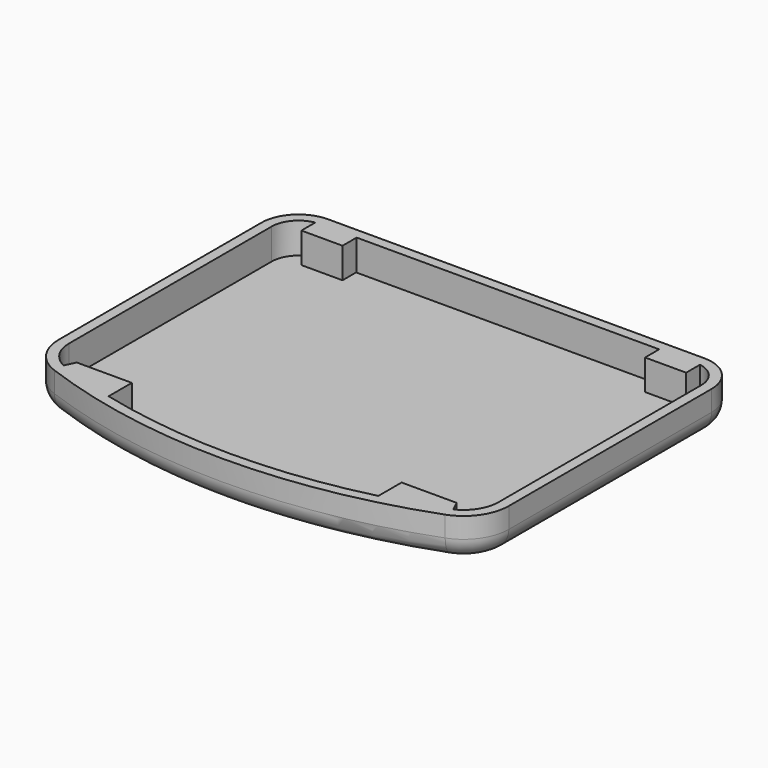
from build123d import *

# Parameters (mm, degrees)
F1_DEPTH = 12.7
F2_T     = -3.175
F3_R     = 6.35
F5_W     = 12.7
F5_H     = 6.35
F6_DEPTH = 9.398


# Not quite as in the source:
# - a feature names something its author has since deleted; it is built from what else it names


with BuildPart() as f1:
    # F0 (on Top) → F1 (new body)
    with BuildSketch(Plane.XY):
        with BuildLine():
            Line((58.0965084505, 62.5356453779), (-58.0965084505, 62.5356453779))
            ThreePointArc((-58.0965084505, 62.5356453779), (-66.1787389595, 59.1878758868), (-69.5265084505, 51.1056453779))
            Line((-69.5265084505, 51.1056453779), (-69.5265084505, -27.1992570698))
            ThreePointArc((-69.5265084505, -27.1992570698), (-67.0115325937, -35.1957139026), (-60.3721316603, -40.3130159932))
            ThreePointArc((-60.3721316603, -40.3130159932), (0, -51.0474727306), (60.3721316603, -40.3130159932))
            ThreePointArc((60.3721316603, -40.3130159932), (67.0115325937, -35.1957139026), (69.5265084505, -27.1992570698))
            Line((69.5265084505, -27.1992570698), (69.5265084505, 51.1056453779))
            ThreePointArc((69.5265084505, 51.1056453779), (66.1787389595, 59.1878758868), (58.0965084505, 62.5356453779))
        make_face()
    extrude(amount=F1_DEPTH)

    # F2
    f2_openings = [f1.faces().sort_by_distance(p)[0] for p in [
        (0, 7.919531, 12.7),
    ]]
    offset(amount=F2_T, openings=f2_openings)

    # F3
    f3_edges = [f1.edges().sort_by_distance(p)[0] for p in [
        (69.526508, 11.953194, 0),
        (66.178739, 59.187876, 0),
        (0, 62.535645, 0),
        (-66.178739, 59.187876, 0),
        (-69.526508, 11.953194, 0),
        (-67.011533, -35.195714, 0),
        (0, -51.047473, 0),
        (67.011533, -35.195714, 0),
    ]]
    fillet(f3_edges, radius=F3_R)

    # F5 (on offset) → F6 (join)
    with BuildSketch(Plane.XY.offset(12.7)):
        with Locations((-53.0805146158, 57.0815077901)):
            Rectangle(F5_W, F5_H)
        with Locations((53.0805146158, 57.0815077901)):
            Rectangle(F5_W, F5_H)
        Polygon((-41.6677072644, -33.773638308), (-58.6946308613, -33.773638308), (-60.6418885291, -37.9110425711), (-53.9016760886, -40.266495198), (-41.6677072644, -43.4330925345), align=None)
        Polygon((60.6418885291, -37.9110425711), (58.6946308613, -33.773638308), (41.6677072644, -33.773638308), (41.6677072644, -43.4330925345), (53.9016760886, -40.266495198), align=None)
    extrude(amount=-F6_DEPTH)


solid = f1.part
